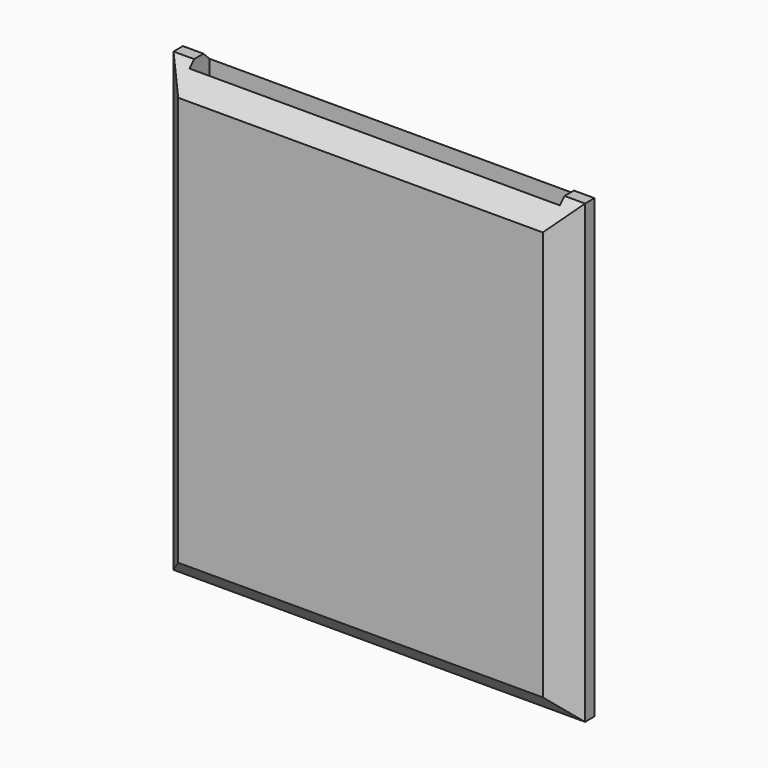
from build123d import *

# Parameters (mm, degrees)
F0_W        = 88.9418646693
F0_H        = 98.6094549298
F1_DEPTH    = 12.7
F2_W        = 80.0476707518
F2_H        = 5.413854029
F3_DEPTH    = 76.2
F4_T1_DEPTH = 124.7377540876
F4_T3_DEPTH = 115.0701638271


# Not quite as in the source:
# - a fillet or chamfer that OpenCascade refuses, or shapes differently, is made with other operations: its cross-section is extruded or revolved along the edge and cut away or added


with BuildPart() as f1:
    # F0 (on Front) → F1 (new body)
    with BuildSketch(Plane.XZ):
        Rectangle(F0_W, F0_H)
    extrude(amount=F1_DEPTH)

    # F2 (on face) → F3 (cut)
    with BuildSketch(Plane.XY.offset(49.3047274649)):
        with Locations((-1.8626e-06, -6.1872594524)):
            Rectangle(F2_W, F2_H)
    extrude(amount=-F3_DEPTH, mode=Mode.SUBTRACT)

    # F4: chamfer of 5.08 on 8 edges, made by hand

    # F4_s2 → F4_t1 (cut)
    with BuildSketch(Plane.XY.offset(-62.3688770438)):
        Polygon((44.4709323347, -5.08), (39.3909323347, 0), (44.4709323347, 0), align=None)
        Polygon((-39.3909323347, 0), (-44.4709323347, -5.08), (-44.4709323347, 0), align=None)
        Polygon((44.4709323347, -7.62), (39.3909323347, -12.7), (44.4709323347, -12.7), align=None)
        Polygon((-39.3909323347, -12.7), (-44.4709323347, -7.62), (-44.4709323347, -12.7), align=None)
    extrude(amount=F4_T1_DEPTH, mode=Mode.SUBTRACT)

    # F4_s4 → F4_t3 (cut)
    with BuildSketch(Plane.YZ.offset(-57.5350819135)):
        Polygon((-5.08, 49.3047274649), (0, 44.2247274649), (0, 49.3047274649), align=None)
        Polygon((-5.08, -49.3047274649), (0, -44.2247274649), (0, -49.3047274649), align=None)
        Polygon((-7.62, 49.3047274649), (-12.7, 44.2247274649), (-12.7, 49.3047274649), align=None)
        Polygon((-7.62, -49.3047274649), (-12.7, -44.2247274649), (-12.7, -49.3047274649), align=None)
    extrude(amount=F4_T3_DEPTH, mode=Mode.SUBTRACT)


solid = f1.part
